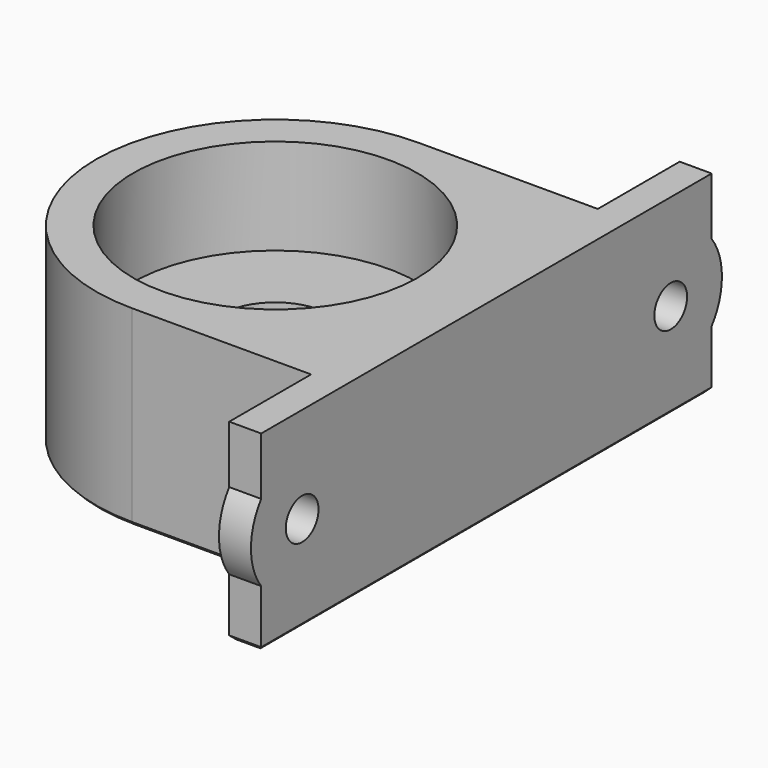
from build123d import *

# Parameters (mm, degrees)
F0_R     = 11.1
F1_DEPTH = 7.5
F0_R_2   = 4.25
F2_DEPTH = 7.5
F3_R     = 1.6
F4_DEPTH = 30.501
F5_SIZE  = 0.3
F6_DEPTH = 2.5


with BuildPart() as f1:
    # F0 (on Top) → F1 (new body)
    with BuildSketch(Plane.XY):
        with BuildLine():
            ThreePointArc((0, -14), (9.8994949366, -9.8994949366), (14, 0))
            ThreePointArc((14, 0), (9.8994949366, 9.8994949366), (0, 14))
            ThreePointArc((0, 14), (-14, 0), (0, -14))
        make_face()
        Circle(F0_R, mode=Mode.SUBTRACT)
        with BuildLine():
            ThreePointArc((0, 14), (9.8994949366, 9.8994949366), (14, 0))
            ThreePointArc((14, 0), (9.8994949366, -9.8994949366), (0, -14))
            Line((0, -14), (14, -14))
            Line((14, -14), (14, -22))
            Line((14, -22), (16.5, -22))
            Line((16.5, -22), (16.5, 0))
            Line((16.5, 0), (16.5, 22))
            Line((16.5, 22), (14, 22))
            Line((14, 22), (14, 14))
            Line((14, 14), (0, 14))
        make_face()
    extrude(amount=F1_DEPTH)

    # F0 (on Top) → F2 (join)
    with BuildSketch(Plane.XY):
        with BuildLine():
            ThreePointArc((0, 14), (9.8994949366, 9.8994949366), (14, 0))
            ThreePointArc((14, 0), (9.8994949366, -9.8994949366), (0, -14))
            Line((0, -14), (14, -14))
            Line((14, -14), (14, -22))
            Line((14, -22), (16.5, -22))
            Line((16.5, -22), (16.5, 0))
            Line((16.5, 0), (16.5, 22))
            Line((16.5, 22), (14, 22))
            Line((14, 22), (14, 14))
            Line((14, 14), (0, 14))
        make_face()
        with BuildLine():
            ThreePointArc((0, -14), (9.8994949366, -9.8994949366), (14, 0))
            ThreePointArc((14, 0), (9.8994949366, 9.8994949366), (0, 14))
            ThreePointArc((0, 14), (-14, 0), (0, -14))
        make_face()
        Circle(F0_R, mode=Mode.SUBTRACT)
        Circle(F0_R)
        Circle(F0_R_2, mode=Mode.SUBTRACT)
    extrude(amount=-F2_DEPTH)

    # F3 (on face) → F4 (cut, through all)
    with BuildSketch(Plane.YZ.offset(16.5)):
        with Locations((18, 0)):
            Circle(F3_R)
        with Locations((-18, 0)):
            Circle(F3_R)
    extrude(amount=-F4_DEPTH, mode=Mode.SUBTRACT)

    # F5
    f5_edges = [f1.edges().sort_by_distance(p)[0] for p in [
        (7, -14, -7.5),
        (14, -18, -7.5),
        (15.25, -22, -7.5),
        (16.5, 0, -7.5),
        (15.25, 22, -7.5),
        (14, 18, -7.5),
        (7, 14, -7.5),
        (-14, 0, -7.5),
        (-4.25, 0, -7.5),
    ]]
    chamfer(f5_edges, length=F5_SIZE)

    # F3 (on face) → F6 (join, through all)
    with BuildSketch(Plane.YZ.offset(16.5)):
        with BuildLine():
            ThreePointArc((22, -3), (22.7434164903, -1.5811388301), (23, 0))
            ThreePointArc((23, 0), (22.7434164903, 1.5811388301), (22, 3))
            Line((22, 3), (22, -3))
        make_face()
        with BuildLine():
            Line((22, -3), (22, 3))
            ThreePointArc((22, 3), (13, 0), (22, -3))
        make_face()
        with Locations((18, 0)):
            Circle(F3_R, mode=Mode.SUBTRACT)
        with BuildLine():
            Line((-22, -3), (-22, 3))
            ThreePointArc((-22, 3), (-23, 0), (-22, -3))
        make_face()
    extrude(amount=-F6_DEPTH)


solid = f1.part
